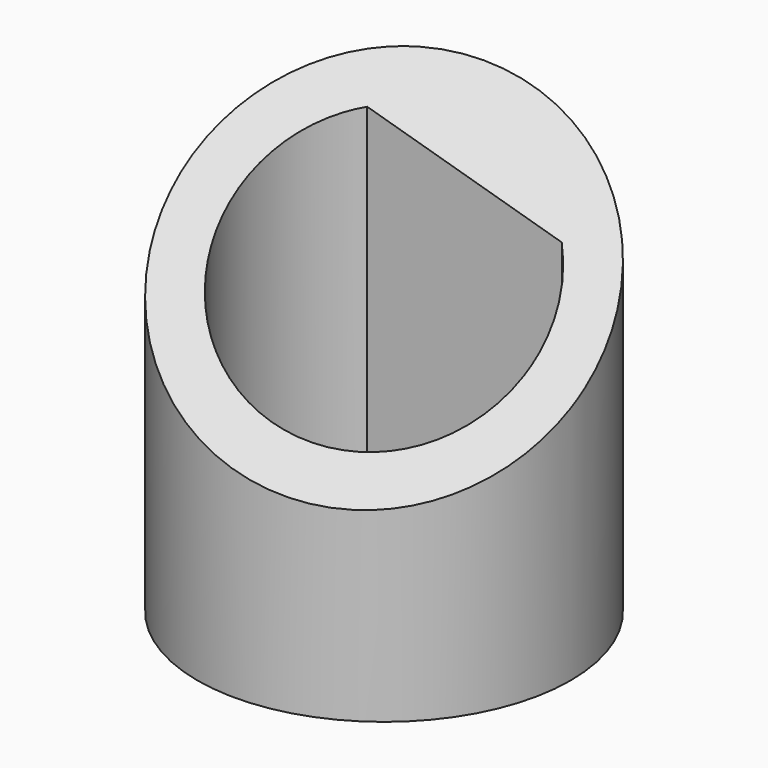
from build123d import *

# Parameters (mm, degrees)
F0_R     = 6
F1_DEPTH = 15
F6_DEPTH = 12.5


# Not quite as in the source:
# - the program builds the solid bodies; features that only make, move or delete a surface that nothing else refers to are left out


with BuildPart() as f1:
    # F0 (on Top) → F1 (new body)
    with BuildSketch(Plane.XY):
        Circle(F0_R)
        with BuildLine():
            ThreePointArc((3.1279784422, 3.2350812764), (4.1428192689, 1.7569998592), (4.5, 0))
            ThreePointArc((4.5, 0), (-1.7569998592, -4.1428192689), (-3.1279784422, 3.2350812764))
            ThreePointArc((-3.1279784422, 3.2350812764), (0, 4.5), (3.1279784422, 3.2350812764))
        make_face(mode=Mode.SUBTRACT)
        with BuildLine():
            Line((-3.1279784422, 3.2350812764), (3.1279784422, 3.2350812764))
            ThreePointArc((3.1279784422, 3.2350812764), (0, 4.5), (-3.1279784422, 3.2350812764))
        make_face()
    extrude(amount=F1_DEPTH)

    # F5 (on face) → F6 (cut, symmetric)
    with BuildSketch(Plane(origin=(0, 0, 0), x_dir=(0.5, -0.8660254038, 0), z_dir=(-0.8660254038, -0.5, 0))):
        Polygon((6.8078478798, 15), (-6, 15), (-6, 12.9036288413), (6.8078478798, 5.5090144201), align=None)
    extrude(amount=F6_DEPTH, both=True, mode=Mode.SUBTRACT)


solid = f1.part
